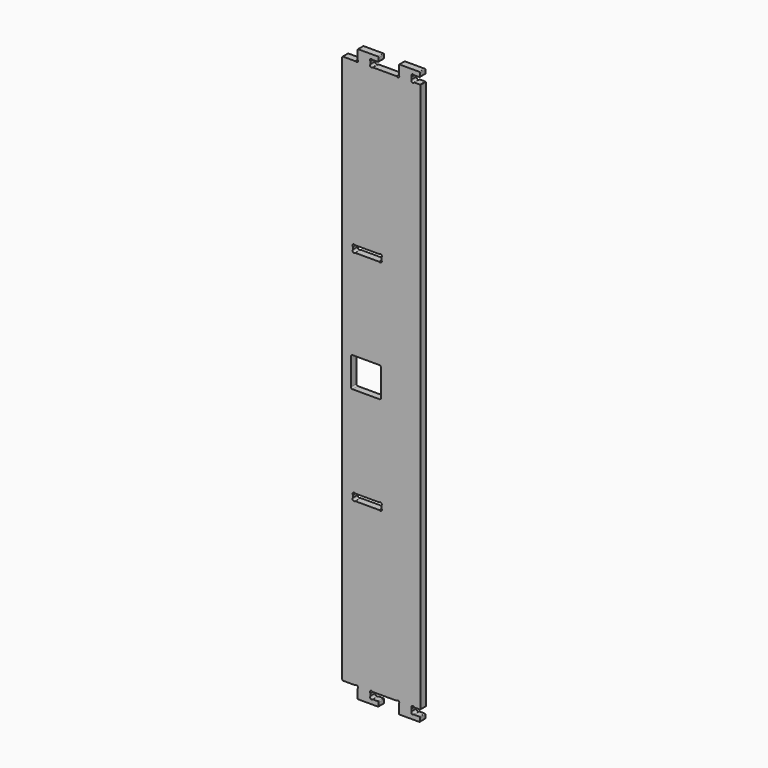
from build123d import *

# Parameters (mm, degrees)
F1_DEPTH = 18


# Not quite as in the source:
# - ends of sketch curves that miss each other by under 0.0002 mm in the source are joined


with BuildPart() as f1:
    # F0 (on Front) → F1 (new body)
    with BuildSketch(Plane.XZ):
        with BuildLine():
            ThreePointArc((-111.5625776076, -719.3076212806), (-111.5625776076, -713.6507670312), (-105.9057233581, -713.6507670312))
            Line((-105.9057233581, -713.6507670312), (-105.2886944829, -714.1507671559))
            Line((-105.2886944829, -714.1507671559), (-41.9563794829, -714.1507671559))
            Line((-41.9563794829, -714.1507671559), (-41.4683634829, -713.6507671559))
            ThreePointArc((-41.4683634829, -713.6507671559), (-35.8115093581, -713.6507670312), (-35.8115093581, -719.3076212806))
            Line((-35.8115093581, -719.3076212806), (-35.8094664829, -742.1509261559))
            ThreePointArc((-35.8094664829, -742.1509261559), (-35.2236167578, -743.5650240029), (-33.8094664829, -744.1507471559))
            Line((-33.8094664829, -744.1507471559), (18.4384905171, -744.1507471559))
            ThreePointArc((18.4384905171, -744.1507471559), (19.8527040795, -743.5649607183), (20.4384905171, -742.1507471559))
            Line((20.4384905171, -742.1507471559), (20.4384905171, -733.6507671559))
            ThreePointArc((20.4384905171, -733.6507671559), (19.8527040795, -732.2365535935), (18.4384905171, -731.6507671559))
            Line((18.4384905171, -731.6507671559), (4.0953445171, -731.6507671559))
            ThreePointArc((4.0953445171, -731.6507671559), (-1.5615098576, -731.6507670306), (-1.5615091076, -725.9939125312))
            Line((-1.5615091076, -725.9939125312), (-1.5615094829, -719.3076211559))
            ThreePointArc((-1.5615094829, -719.3076211559), (-1.5615096076, -713.6507670312), (4.0953446419, -713.6507670312))
            Line((4.0953446419, -713.6507670312), (5.0690155171, -714.6507671559))
            Line((5.0690155171, -714.6507671559), (20.4374225171, -714.6507671559))
            ThreePointArc((20.4374225171, -714.6507671559), (21.1445292983, -714.3578739371), (21.4374225171, -713.6507671559))
            Line((21.4374225171, -713.6507671559), (21.4374225171, 749.3492328441))
            ThreePointArc((21.4374225171, 749.3492328441), (21.1445292983, 750.0563396253), (20.4374225171, 750.3492328441))
            Line((20.4374225171, 750.3492328441), (5.1226495171, 750.3492328441))
            Line((5.1226495171, 750.3492328441), (4.0953445171, 749.3492328441))
            ThreePointArc((4.0953445171, 749.3492328441), (-1.5615098576, 749.3492329694), (-1.5615091076, 755.0060874688))
            Line((-1.5615091076, 755.0060874688), (-1.5615094829, 761.6923788441))
            ThreePointArc((-1.5615094829, 761.6923788441), (-1.5615096076, 767.3492329688), (4.0953446419, 767.3492329688))
            Line((4.0953446419, 767.3492329688), (18.4384905171, 767.3492328441))
            ThreePointArc((18.4384905171, 767.3492328441), (19.8527040795, 767.9350192817), (20.4384905171, 769.3492328441))
            Line((20.4384905171, 769.3492328441), (20.4384905171, 777.8492138441))
            ThreePointArc((20.4384905171, 777.8492138441), (19.8527040795, 779.2634274065), (18.4384905171, 779.8492138441))
            Line((18.4384905171, 779.8492138441), (-33.8094664829, 779.8492138441))
            ThreePointArc((-33.8094664829, 779.8492138441), (-35.2236171114, 779.2634903376), (-35.809466475, 777.8493918441))
            Line((-35.809466475, 777.8493918441), (-35.8115094829, 755.0060878441))
            ThreePointArc((-35.8115094829, 755.0060878441), (-35.8115091081, 749.3492329694), (-41.4683636076, 749.3492327194))
            Line((-41.4683636076, 749.3492327194), (-41.9683634829, 749.8492328441))
            Line((-41.9683634829, 749.8492328441), (-105.2468454829, 749.8492328441))
            Line((-105.2468454829, 749.8492328441), (-105.9057234829, 749.3492328441))
            ThreePointArc((-105.9057234829, 749.3492328441), (-111.5625778576, 749.3492329694), (-111.5625771076, 755.0060874688))
            Line((-111.5625771076, 755.0060874688), (-111.5625774829, 761.6923788441))
            ThreePointArc((-111.5625774829, 761.6923788441), (-111.5625776076, 767.3492329688), (-105.9057233581, 767.3492329688))
            Line((-105.9057233581, 767.3492329688), (-91.5625774829, 767.3492328441))
            ThreePointArc((-91.5625774829, 767.3492328441), (-90.1483639205, 767.9350192817), (-89.5625774829, 769.3492328441))
            Line((-89.5625774829, 769.3492328441), (-89.5625774829, 777.8492138441))
            ThreePointArc((-89.5625774829, 777.8492138441), (-90.1483639205, 779.2634274065), (-91.5625774829, 779.8492138441))
            Line((-91.5625774829, 779.8492138441), (-143.8105344829, 779.8492138441))
            ThreePointArc((-143.8105344829, 779.8492138441), (-145.2246851114, 779.2634903376), (-145.810534475, 777.8493918441))
            Line((-145.810534475, 777.8493918441), (-145.8125774829, 755.0060878441))
            ThreePointArc((-145.8125774829, 755.0060878441), (-145.8125771081, 749.3492329694), (-151.4694316076, 749.3492327194))
            Line((-151.4694316076, 749.3492327194), (-184.5625764829, 749.3492328441))
            ThreePointArc((-184.5625764829, 749.3492328441), (-185.9767900453, 748.7634464065), (-186.5625764829, 747.3492328441))
            Line((-186.5625764829, 747.3492328441), (-186.5625764829, -711.6507671559))
            ThreePointArc((-186.5625764829, -711.6507671559), (-185.9767900453, -713.0649807183), (-184.5625764829, -713.6507671559))
            Line((-184.5625764829, -713.6507671559), (-151.4694314829, -713.6507671559))
            ThreePointArc((-151.4694314829, -713.6507671559), (-145.8125773581, -713.6507670312), (-145.8125773581, -719.3076212806))
            Line((-145.8125773581, -719.3076212806), (-145.8105344829, -742.1509261559))
            ThreePointArc((-145.8105344829, -742.1509261559), (-145.2246847578, -743.5650240029), (-143.8105344829, -744.1507471559))
            Line((-143.8105344829, -744.1507471559), (-91.5625774829, -744.1507471559))
            ThreePointArc((-91.5625774829, -744.1507471559), (-90.1483639205, -743.5649607183), (-89.5625774829, -742.1507471559))
            Line((-89.5625774829, -742.1507471559), (-89.5625774829, -733.6507671559))
            ThreePointArc((-89.5625774829, -733.6507671559), (-90.1483639205, -732.2365535935), (-91.5625774829, -731.6507671559))
            Line((-91.5625774829, -731.6507671559), (-105.9057234829, -731.6507671559))
            ThreePointArc((-105.9057234829, -731.6507671559), (-111.5625778576, -731.6507670306), (-111.5625771076, -725.9939125312))
            Line((-111.5625771076, -725.9939125312), (-111.5625776076, -719.3076212806))
        make_face()
        with BuildLine():
            ThreePointArc((-82.3041508581, -276.4939125312), (-82.3041501081, -282.1507670306), (-87.9610046076, -282.1507672806))
            Line((-87.9610046076, -282.1507672806), (-152.4757234829, -282.1507671559))
            ThreePointArc((-152.4757234829, -282.1507671559), (-158.1325778576, -282.1507670306), (-158.1325771076, -276.4939125312))
            Line((-158.1325771076, -276.4939125312), (-158.1325774829, -269.8076211559))
            ThreePointArc((-158.1325774829, -269.8076211559), (-158.1325776076, -264.1507670312), (-152.4757233581, -264.1507670312))
            Line((-152.4757233581, -264.1507670312), (-87.9610044829, -264.1507671559))
            ThreePointArc((-87.9610044829, -264.1507671559), (-82.3041503581, -264.1507670312), (-82.3041503581, -269.8076212806))
            Line((-82.3041503581, -269.8076212806), (-82.3041508581, -276.4939125312))
        make_face(mode=Mode.SUBTRACT)
        with BuildLine():
            Line((-163.4866634829, -18.1507671559), (-163.4866634829, 53.8492328441))
            ThreePointArc((-163.4866634829, 53.8492328441), (-162.3150906076, 56.6776599688), (-159.4866634829, 57.8492328441))
            Line((-159.4866634829, 57.8492328441), (-87.4866634829, 57.8492328441))
            ThreePointArc((-87.4866634829, 57.8492328441), (-84.6582363581, 56.6776599688), (-83.4866634829, 53.8492328441))
            Line((-83.4866634829, 53.8492328441), (-83.4866634829, -18.1507671559))
            ThreePointArc((-83.4866634829, -18.1507671559), (-84.6582363581, -20.9791942806), (-87.4866634829, -22.1507671559))
            Line((-87.4866634829, -22.1507671559), (-159.4866634829, -22.1507671559))
            ThreePointArc((-159.4866634829, -22.1507671559), (-162.3150906076, -20.9791942806), (-163.4866634829, -18.1507671559))
        make_face(mode=Mode.SUBTRACT)
        with BuildLine():
            Line((-82.3041504829, 312.1923788441), (-82.3041504829, 305.5060878441))
            ThreePointArc((-82.3041504829, 305.5060878441), (-82.3041503581, 299.8492327194), (-87.9610046076, 299.8492327194))
            Line((-87.9610046076, 299.8492327194), (-152.4757234829, 299.8492328441))
            ThreePointArc((-152.4757234829, 299.8492328441), (-158.1325778576, 299.8492329694), (-158.1325771076, 305.5060874688))
            Line((-158.1325771076, 305.5060874688), (-158.1325774829, 312.1923788441))
            ThreePointArc((-158.1325774829, 312.1923788441), (-158.1325776076, 317.8492329688), (-152.4757233581, 317.8492329688))
            Line((-152.4757233581, 317.8492329688), (-87.9610044829, 317.8492328441))
            ThreePointArc((-87.9610044829, 317.8492328441), (-82.3041503581, 317.8492329688), (-82.3041504829, 312.1923788441))
        make_face(mode=Mode.SUBTRACT)
    extrude(amount=-F1_DEPTH)


solid = f1.part
